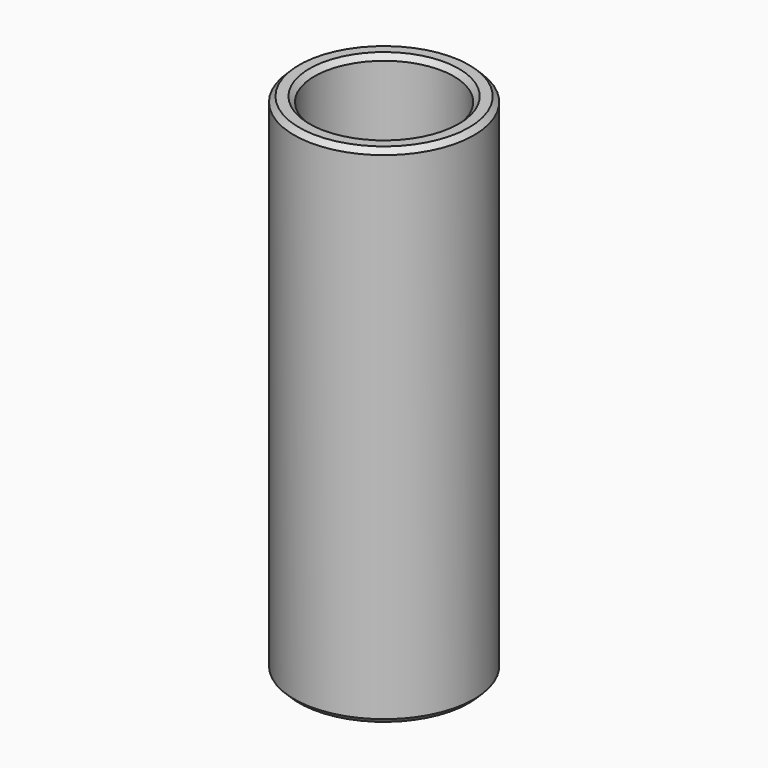
from build123d import *

# Parameters (mm, degrees)
F0_R     = 7.1
F0_R_2   = 5.5
F1_DEPTH = 40
F2_START = 19.8
F0_R_3   = 5.1
F2_DEPTH = 0.4
F3_SIZE  = 0.39999
F4_SIZE  = 0.4


# Not quite as in the source:
# - a fillet or chamfer is up to 0.001 mm smaller than in the source, because OpenCascade refuses the exact size


with BuildPart() as f1:
    # F0 (on Top) → F1 (new body)
    with BuildSketch(Plane.XY):
        Circle(F0_R)
        Circle(F0_R_2, mode=Mode.SUBTRACT)
    extrude(amount=F1_DEPTH)

    # F0 (on Top) → F2 (join)
    with BuildSketch(Plane.XY.offset(F2_START)):
        Circle(F0_R_2)
        Circle(F0_R_3, mode=Mode.SUBTRACT)
    extrude(amount=F2_DEPTH)

    # F3 (size 0.4 in the source; OpenCascade refuses exactly that, so slightly less here)
    f3_edges = [f1.edges().sort_by_distance(p)[0] for p in [
        (-5.5, 0, 19.8),
        (-5.5, 0, 20.2),
    ]]
    chamfer(f3_edges, length=F3_SIZE)

    # F4
    f4_edges = [f1.edges().sort_by_distance(p)[0] for p in [
        (-5.5, 0, 40),
        (-7.1, 0, 40),
        (-5.5, 0, 0),
        (-7.1, 0, 0),
    ]]
    chamfer(f4_edges, length=F4_SIZE)


solid = f1.part
